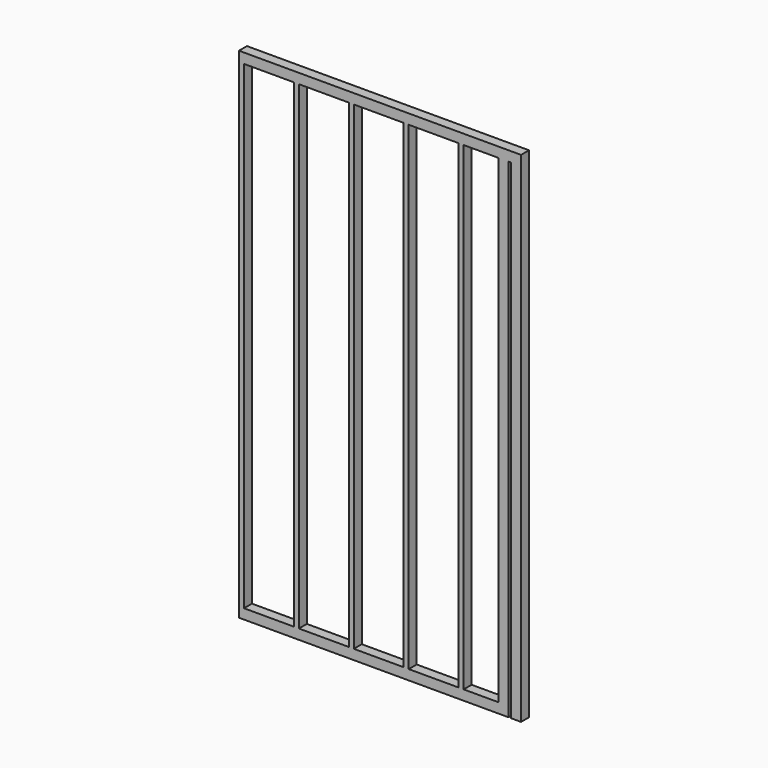
from build123d import *

# Parameters (mm, degrees)
F0_W      = 12.7
F0_H      = 1219.2
F1_DEPTH  = 25.4
F2_W      = 406.4
F2_H      = 1396.9661742449
F2_W_2    = 69.85
F2_H_2    = 1270
F2_W_3    = 63.5
F3_DEPTH  = 25.4
F4_W      = 25.4
F4_H      = 1270
F5_DEPTH  = 25.4
F6_W      = 25.4
F6_H      = 1270
F7_DEPTH  = 25.4
F6_H_2    = 25.4
F6_W_2    = 31.75
F6_H_3    = 1244.6
F9_W      = 975.7457971573
F9_H      = 1423.7642139196
F10_DEPTH = 218.67692


with BuildPart() as f1:
    # F0 (on Front) → F1 (new body)
    with BuildSketch(Plane.XZ):
        Polygon((-930.275, 1270), (-930.275, 1244.6), (-771.525, 1244.6), (-758.825, 1244.6), (-631.825, 1244.6), (-619.125, 1244.6), (-492.125, 1244.6), (-479.425, 1244.6), (-352.425, 1244.6), (-339.725, 1244.6), (-212.725, 1244.6), (-200.025, 1244.6), (-73.025, 1244.6), (-60.325, 1244.6), (66.675, 1244.6), (79.375, 1244.6), (206.375, 1244.6), (219.075, 1244.6), (346.075, 1244.6), (358.775, 1244.6), (485.775, 1244.6), (498.475, 1244.6), (625.475, 1244.6), (638.175, 1244.6), (765.175, 1244.6), (777.875, 1244.6), (930.275, 1244.6), (930.275, 1270), align=None)
        with Locations((-765.175, 635)):
            Rectangle(F0_W, F0_H)
        Polygon((-758.825, 25.4), (-771.525, 25.4), (-930.275, 25.4), (-930.275, 0), (930.275, 0), (930.275, 25.4), (777.875, 25.4), (765.175, 25.4), (638.175, 25.4), (625.475, 25.4), (498.475, 25.4), (485.775, 25.4), (358.775, 25.4), (346.075, 25.4), (219.075, 25.4), (206.375, 25.4), (79.375, 25.4), (66.675, 25.4), (-60.325, 25.4), (-73.025, 25.4), (-200.025, 25.4), (-212.725, 25.4), (-339.725, 25.4), (-352.425, 25.4), (-479.425, 25.4), (-492.125, 25.4), (-619.125, 25.4), (-631.825, 25.4), align=None)
        with Locations((771.525, 635)):
            Rectangle(F0_W, F0_H)
        with Locations((-625.475, 635)):
            Rectangle(F0_W, F0_H)
        with Locations((-485.775, 635)):
            Rectangle(F0_W, F0_H)
        with Locations((-346.075, 635)):
            Rectangle(F0_W, F0_H)
        with Locations((-206.375, 635)):
            Rectangle(F0_W, F0_H)
        with Locations((-66.675, 635)):
            Rectangle(F0_W, F0_H)
        with Locations((73.025, 635)):
            Rectangle(F0_W, F0_H)
        with Locations((212.725, 635)):
            Rectangle(F0_W, F0_H)
        with Locations((352.425, 635)):
            Rectangle(F0_W, F0_H)
        with Locations((492.125, 635)):
            Rectangle(F0_W, F0_H)
        with Locations((631.825, 635)):
            Rectangle(F0_W, F0_H)
    extrude(amount=F1_DEPTH)

    # F2 (on face) → F3 (cut)
    with BuildSketch(Plane.XZ.offset(25.4)):
        with Locations((3.175, 593.5398563743)):
            Rectangle(F2_W, F2_H)
        with Locations((-895.35, 635)):
            Rectangle(F2_W_2, F2_H_2)
        with Locations((898.525, 635)):
            Rectangle(F2_W_3, F2_H_2)
    extrude(amount=-F3_DEPTH, mode=Mode.SUBTRACT)

    # F4 (on face) → F5, piece 2 (join)
    with BuildSketch(Plane.XZ.offset(25.4)):
        with Locations((879.475, 635)):
            Rectangle(F4_W, F4_H)
    extrude(amount=-F5_DEPTH)

    # F6 (on face) → F7, piece 2 (join)
    with BuildSketch(Plane.XZ.offset(25.4)):
        with Locations((911.225, 1257.3)):
            Rectangle(F6_W, F6_H_2)
        with Locations((882.65, 1257.3)):
            Rectangle(F6_W_2, F6_H_2)
        with Locations((911.225, 622.3)):
            Rectangle(F6_W, F6_H_3)
    extrude(amount=-F7_DEPTH)

    # F8: union 


with BuildPart() as f5:
    # F4 (on face) → F5 (new body)
    with BuildSketch(Plane.XZ.offset(25.4)):
        with Locations((-873.125, 635)):
            Rectangle(F4_W, F4_H)
    extrude(amount=-F5_DEPTH)


with BuildPart() as f7:
    # F6 (on face) → F7 (new body)
    with BuildSketch(Plane.XZ.offset(25.4)):
        with Locations((-904.875, 635)):
            Rectangle(F6_W, F6_H)
    extrude(amount=-F7_DEPTH)


with BuildPart() as f10_tool:
    # F9 (on face) → F10 (new body)
    with BuildSketch(Plane(origin=(0, 0, 0), x_dir=(-1, 0, 0), z_dir=(0, 1, 0))):
        with Locations((666.6726469994, 601.2135818601)):
            Rectangle(F9_W, F9_H)
    extrude(amount=-F10_DEPTH)


with BuildPart() as f1_1:
    add(f1.part)

    # F10: cut by f10_tool
    add(f10_tool.part, mode=Mode.SUBTRACT)


with BuildPart() as f5_1:
    add(f5.part)

    # F10: cut by f10_tool
    add(f10_tool.part, mode=Mode.SUBTRACT)


with BuildPart() as f7_1:
    add(f7.part)

    # F10: cut by f10_tool
    add(f10_tool.part, mode=Mode.SUBTRACT)


solid = f1_1.part
